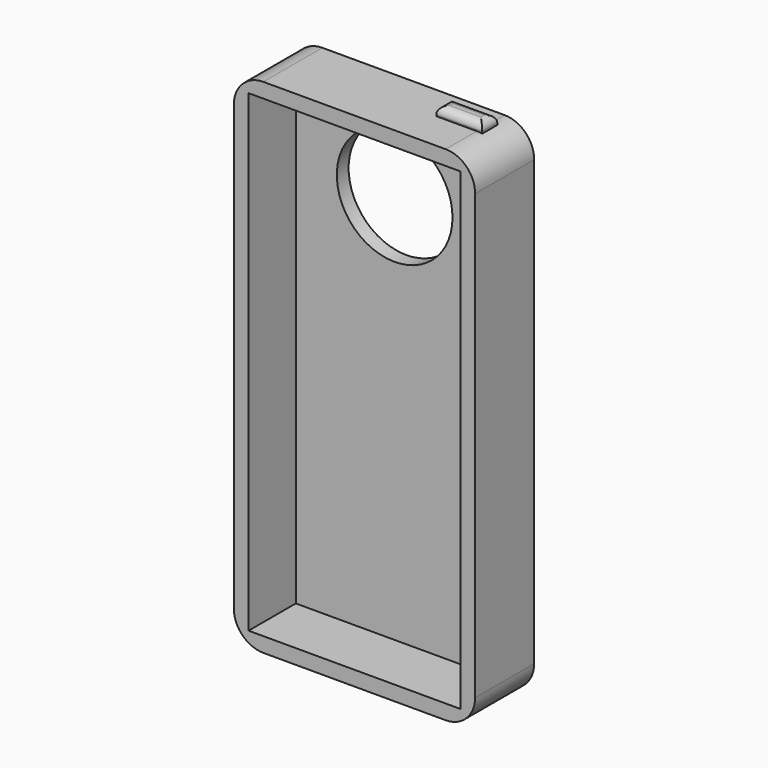
from build123d import *

# Parameters (mm, degrees)
F0_W          = 41.536912322
F0_H          = 86.5394547582
F1_DEPTH      = 12.7
F2_T          = -2.54
F3_R          = 2.2759132083
F5_DEPTH      = 1.524
F4_R          = 2.2733
F6_DEPTH      = 1.524
F7_W          = 7.9097328708
F7_H          = 3.2450191211
F8_DEPTH      = 1.524
F9_R          = 1.27
F10_R         = 5.08
F11_R         = 5.08
F12_T4_DEPTH  = 38.1
F12_T10_DEPTH = 38.1
F12_T16_DEPTH = 38.1
F12_T23_DEPTH = 38.1
F12_T29_DEPTH = 38.1
F13_R         = 5.08
F14_R         = 3.4214532803
F15_DEPTH     = 37.77729
F16_R         = 9.955312615
F17_DEPTH     = 26.73123


# Not quite as in the source:
# - a fillet or chamfer that OpenCascade refuses, or shapes differently, is made with other operations: its cross-section is extruded or revolved along the edge and cut away or added


with BuildPart() as f1:
    # F0 (on Front) → F1 (new body)
    with BuildSketch(Plane.XZ):
        with Locations((-20.768456161, -43.2697273791)):
            Rectangle(F0_W, F0_H)
    extrude(amount=F1_DEPTH)

    # F2
    f2_openings = [f1.faces().sort_by_distance(p)[0] for p in [
        (-20.768456, -12.7, -43.269727),
    ]]
    offset(amount=F2_T, openings=f2_openings)

    # F3 (on face) → F5 (join)
    with BuildSketch(Plane(origin=(-41.536912322, 0, 0), x_dir=(0, -1, 0), z_dir=(-1, 0, 0))):
        with Locations((4.2136539705, -15.7545246184)):
            Circle(F3_R)
    extrude(amount=F5_DEPTH)

    # F4 (on face) → F6 (join)
    with BuildSketch(Plane(origin=(-41.536912322, 0, 0), x_dir=(0, -1, 0), z_dir=(-1, 0, 0))):
        with Locations((3.8371200208, -24.8998850584)):
            Circle(F4_R)
    extrude(amount=F6_DEPTH)

    # F7 (on face) → F8 (join)
    with BuildSketch(Plane.XY):
        with Locations((-8.1125465222, -4.3604943203)):
            Rectangle(F7_W, F7_H)
    extrude(amount=F8_DEPTH)

    # F9
    f9_edges = [f1.edges().sort_by_distance(p)[0] for p in [
        (-8.112547, -2.737985, 1.524),
        (-12.067413, -4.360494, 1.524),
        (-8.112547, -5.983004, 1.524),
        (-4.15768, -4.360494, 1.524),
    ]]
    fillet(f9_edges, radius=F9_R)

    # F10
    f10_edges = [f1.edges().sort_by_distance(p)[0] for p in [
        (-41.536912, -6.35, 0),
    ]]
    fillet(f10_edges, radius=F10_R)

    # F11
    f11_edges = [f1.edges().sort_by_distance(p)[0] for p in [
        (-41.536912, -6.35, -86.539455),
    ]]
    fillet(f11_edges, radius=F11_R)

    # F12: fillet of radius 5.08 on 1 edges, made by hand


with BuildPart() as f12_tool2:
    # F12_s3 → F12_t4 (new body)
    with BuildSketch(Plane.XZ.offset(-12.7)):
        with BuildLine():
            ThreePointArc((-5.08, 0), (-1.4878975516, -1.4878975516), (0, -5.08))
            Line((0, -5.08), (0, 0))
            Line((0, 0), (-5.08, 0))
        make_face()
    extrude(amount=F12_T4_DEPTH)

    split(bisect_by=Plane.YZ.offset(-4.1576800868), keep=Keep.BOTTOM)

    split(bisect_by=Plane.XZ.offset(2.7379847597), keep=Keep.BOTTOM)


with BuildPart() as f1_1:
    add(f1.part)

    # F12_t1: cut F12_tool2
    add(f12_tool2.part, mode=Mode.SUBTRACT)


with BuildPart() as f12_tool8:
    # F12_s9 → F12_t10 (new body)
    with BuildSketch(Plane.XZ.offset(-12.7)):
        with BuildLine():
            ThreePointArc((-5.08, 0), (-1.4878975516, -1.4878975516), (0, -5.08))
            Line((0, -5.08), (0, 0))
            Line((0, 0), (-5.08, 0))
        make_face()
    extrude(amount=F12_T10_DEPTH)

    split(bisect_by=Plane.YZ.offset(-4.1576800868), keep=Keep.TOP)

    split(bisect_by=Plane.XZ.offset(2.7379847597), keep=Keep.BOTTOM)


with BuildPart() as f1_2:
    add(f1_1.part)

    # F12_t7: cut F12_tool8
    add(f12_tool8.part, mode=Mode.SUBTRACT)


with BuildPart() as f12_tool14:
    # F12_s15 → F12_t16 (new body)
    with BuildSketch(Plane.XZ.offset(-12.7)):
        with BuildLine():
            ThreePointArc((-5.08, 0), (-1.4878975516, -1.4878975516), (0, -5.08))
            Line((0, -5.08), (0, 0))
            Line((0, 0), (-5.08, 0))
        make_face()
    extrude(amount=F12_T16_DEPTH)

    split(bisect_by=Plane.YZ.offset(-4.1576800868), keep=Keep.TOP)

    split(bisect_by=Plane.XZ.offset(5.9830038808), keep=Keep.BOTTOM)

    split(bisect_by=Plane.XZ.offset(2.7379847597), keep=Keep.TOP)


with BuildPart() as f1_3:
    add(f1_2.part)

    # F12_t13: cut F12_tool14
    add(f12_tool14.part, mode=Mode.SUBTRACT)


with BuildPart() as f12_tool21:
    # F12_s22 → F12_t23 (new body)
    with BuildSketch(Plane.XZ.offset(-12.7)):
        with BuildLine():
            ThreePointArc((-5.08, 0), (-1.4878975516, -1.4878975516), (0, -5.08))
            Line((0, -5.08), (0, 0))
            Line((0, 0), (-5.08, 0))
        make_face()
    extrude(amount=F12_T23_DEPTH)

    split(bisect_by=Plane.YZ.offset(-4.1576800868), keep=Keep.BOTTOM)

    split(bisect_by=Plane.XZ.offset(5.9830038808), keep=Keep.TOP)


with BuildPart() as f1_4:
    add(f1_3.part)

    # F12_t20: cut F12_tool21
    add(f12_tool21.part, mode=Mode.SUBTRACT)


with BuildPart() as f12_tool27:
    # F12_s28 → F12_t29 (new body)
    with BuildSketch(Plane.XZ.offset(-12.7)):
        with BuildLine():
            ThreePointArc((-5.08, 0), (-1.4878975516, -1.4878975516), (0, -5.08))
            Line((0, -5.08), (0, 0))
            Line((0, 0), (-5.08, 0))
        make_face()
    extrude(amount=F12_T29_DEPTH)

    split(bisect_by=Plane.YZ.offset(-4.1576800868), keep=Keep.TOP)

    split(bisect_by=Plane.XZ.offset(5.9830038808), keep=Keep.TOP)


with BuildPart() as f1_5:
    add(f1_4.part)

    # F12_t26: cut F12_tool27
    add(f12_tool27.part, mode=Mode.SUBTRACT)

    # F13
    f13_edges = [f1_5.edges().sort_by_distance(p)[0] for p in [
        (0, -6.35, -86.539455),
    ]]
    fillet(f13_edges, radius=F13_R)

    # F14 (on face) → F15 (cut)
    with BuildSketch(Plane(origin=(0, 0, 0), x_dir=(-1, 0, 0), z_dir=(0, 1, 0))):
        with Locations((6.212700624, -10.3420317173)):
            Circle(F14_R)
    extrude(amount=-F15_DEPTH, mode=Mode.SUBTRACT)

    # F16 (on face) → F17 (cut)
    with BuildSketch(Plane.XZ.offset(2.54)):
        with Locations((-21.9822023064, -16.7564060539)):
            Circle(F16_R)
    extrude(amount=-F17_DEPTH, mode=Mode.SUBTRACT)


solid = f1_5.part
